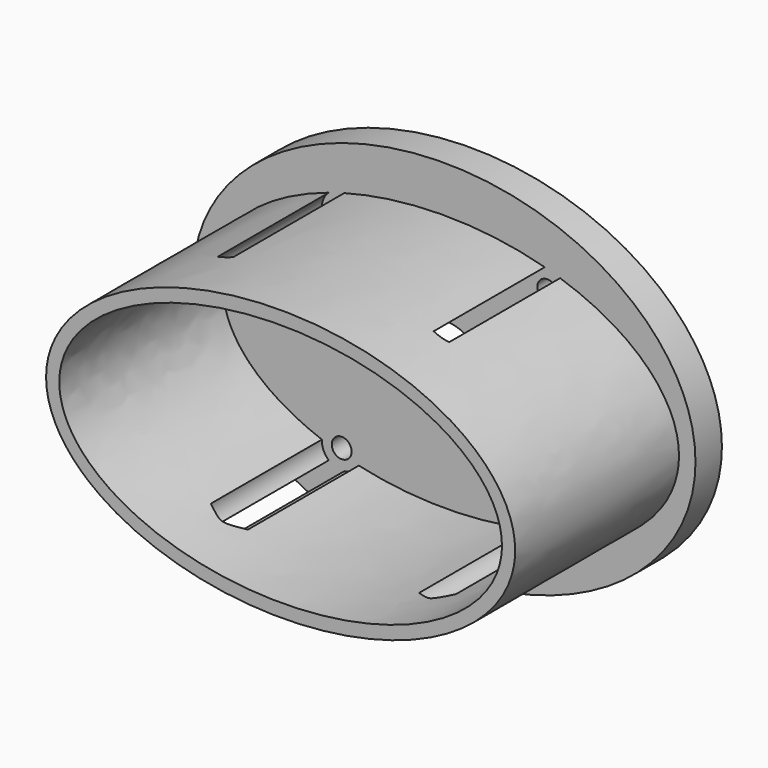
from build123d import *

# Parameters (mm, degrees)
F1_DEPTH = 31
F3_DEPTH = 5
F4_D     = 13
F4_DEPTH = 5
F4_TIP   = 3.9055940237
F6_D     = 3
F6_DEPTH = 5
F6_TIP   = 0.9012909285
F7_D     = 6
F7_DEPTH = 21
F7_TIP   = 1.8025818571


# Not quite as in the source:
# - a feature names something its author has since deleted; it is built from what else it names


with BuildPart() as f1:
    # F0 (on Front) → F1 (new body)
    with BuildSketch(Plane.XZ):
        with BuildLine():
            add(Edge.make_bspline(
                [(35.5, 0), (35.5, 35.5070415552), (-17.75, 17.7535207776), (-71, 0), (-17.75, -17.7535207776), (35.5, -35.5070415552), (35.5, 0)],
                knots=[0, 0, 0, 2.0943951024, 2.0943951024, 4.1887902048, 4.1887902048, 6.2831853072, 6.2831853072, 6.2831853072], degree=2, weights=[1, 0.5, 1, 0.5, 1, 0.5, 1]))
        make_face()
        with BuildLine():
            add(Edge.make_bspline(
                [(33.5, 0), (33.5, 32.04293994), (-16.75, 16.02146997), (-67, 0), (-16.75, -16.02146997), (33.5, -32.04293994), (33.5, 0)],
                knots=[0, 0, 0, 2.0943951024, 2.0943951024, 4.1887902048, 4.1887902048, 6.2831853072, 6.2831853072, 6.2831853072], degree=2, weights=[1, 0.5, 1, 0.5, 1, 0.5, 1]))
        make_face(mode=Mode.SUBTRACT)
    extrude(amount=F1_DEPTH)

    # F2 (on Front) → F3 (join)
    with BuildSketch(Plane.XZ):
        with BuildLine():
            add(Edge.make_bspline(
                [(38, 0), (38, 47.6313972081), (-19, 23.8156986041), (-76, 0), (-19, -23.8156986041), (38, -47.6313972081), (38, 0)],
                knots=[0, 0, 0, 2.0943951024, 2.0943951024, 4.1887902048, 4.1887902048, 6.2831853072, 6.2831853072, 6.2831853072], degree=2, weights=[1, 0.5, 1, 0.5, 1, 0.5, 1]))
        make_face()
    extrude(amount=-F3_DEPTH)

    # F4
    with Locations(Plane.XZ):
        with Locations((0, 0)):
            Hole(F4_D / 2, depth=F4_DEPTH)
            with Locations((0, 0, -(F4_DEPTH + F4_TIP / 2))):  # 118° drill point
                Cone(0, F4_D / 2, F4_TIP, mode=Mode.SUBTRACT)

    # F6 (one way)
    with BuildSketch(Plane.XZ):
        with Locations((-15.5563491861, 15.5563491861), (15.5563491861, 15.5563491861), (-15.5563491861, -15.5563491861), (15.5563491861, -15.5563491861)):
            Circle(F6_D / 2)
    extrude(amount=-F6_DEPTH, mode=Mode.SUBTRACT)
    with Locations(Plane.XZ):
        with Locations((-15.5563491861, 15.5563491861), (15.5563491861, 15.5563491861), (-15.5563491861, -15.5563491861), (15.5563491861, -15.5563491861)):
            with Locations((0, 0, -(F6_DEPTH + F6_TIP / 2))):  # 118° drill point
                Cone(0, F6_D / 2, F6_TIP, mode=Mode.SUBTRACT)

    # F7 (one way)
    with BuildSketch(Plane(origin=(0, 0, 0), x_dir=(1, 0, 0), z_dir=(0, 1, 0))):
        with Locations((-15.5563491861, -15.5563491861), (15.5563491861, -15.5563491861), (15.5563491861, 15.5563491861), (-15.5563491861, 15.5563491861)):
            Circle(F7_D / 2)
    extrude(amount=-F7_DEPTH, mode=Mode.SUBTRACT)
    with Locations(Plane(origin=(0, 0, 0), x_dir=(1, 0, 0), z_dir=(0, 1, 0))):
        with Locations((-15.5563491861, -15.5563491861), (15.5563491861, -15.5563491861), (15.5563491861, 15.5563491861), (-15.5563491861, 15.5563491861)):
            with Locations((0, 0, -(F7_DEPTH + F7_TIP / 2))):  # 118° drill point
                Cone(0, F7_D / 2, F7_TIP, mode=Mode.SUBTRACT)


solid = f1.part
